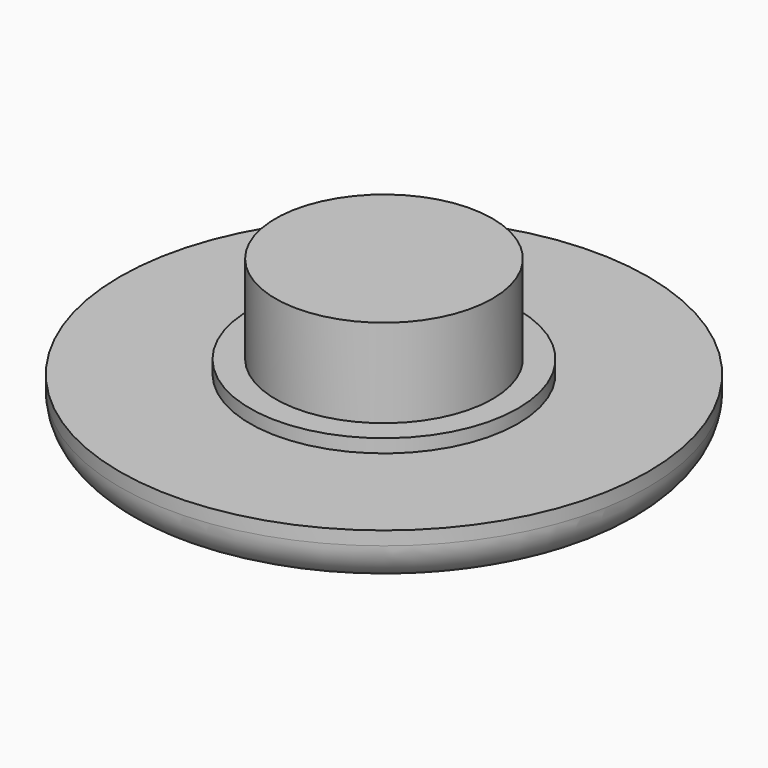
from build123d import *

# Parameters (mm, degrees)
F0_R     = 9.8592181747
F1_DEPTH = 2
F2_R     = 5
F3_DEPTH = 0.5
F4_R     = 4.05
F5_DEPTH = 3.3
F6_R     = 8.5
F7_DEPTH = 1


# Not quite as in the source:
# - a fillet or chamfer that OpenCascade refuses, or shapes differently, is made with other operations: its cross-section is extruded or revolved along the edge and cut away or added


with BuildPart() as f1:
    # F0 (on Top) → F1 (new body)
    with BuildSketch(Plane.XY):
        Circle(F0_R)
    extrude(amount=F1_DEPTH)

    # F2 (on face) → F3 (join)
    with BuildSketch(Plane.XY.offset(2)):
        Circle(F2_R)
    extrude(amount=F3_DEPTH)

    # F4 (on face) → F5 (join)
    with BuildSketch(Plane.XY.offset(2.5)):
        Circle(F4_R)
    extrude(amount=F5_DEPTH)

    # F6 (on face) → F7 (cut)
    with BuildSketch(Plane(origin=(0, 0, 0), x_dir=(1, 0, 0), z_dir=(0, 0, -1))):
        Circle(F6_R)
    extrude(amount=-F7_DEPTH, mode=Mode.SUBTRACT)

    # F8: fillet of radius 32 on 1 edges, made by hand

    # F8_s1 → F8_t2 (revolve)
    with BuildSketch(Plane.XZ):
        with BuildLine():
            ThreePointArc((8.5, 0), (4.5627460668, 0.7490157328), (0.5627460668, 1))
            Line((0.5627460668, 1), (8.5, 1))
            Line((8.5, 1), (8.5, 0))
        make_face()
    revolve(axis=Axis((0, 0, 1), (0, 0, -1)))

    # F9: fillet of radius 1.5 on 1 edges, made by hand

    # F9_s1 → F9_t2 (revolve, cut)
    with BuildSketch(Plane.XZ):
        with BuildLine():
            ThreePointArc((9.8592181747, 1.4933788795), (9.4685361494, 0.4837187233), (8.5, 0))
            Line((8.5, 0), (9.8592181747, 0))
            Line((9.8592181747, 0), (9.8592181747, 1.4933788795))
        make_face()
    revolve(axis=Axis((0, 0, 0), (0, 0, 1)), mode=Mode.SUBTRACT)


solid = f1.part
